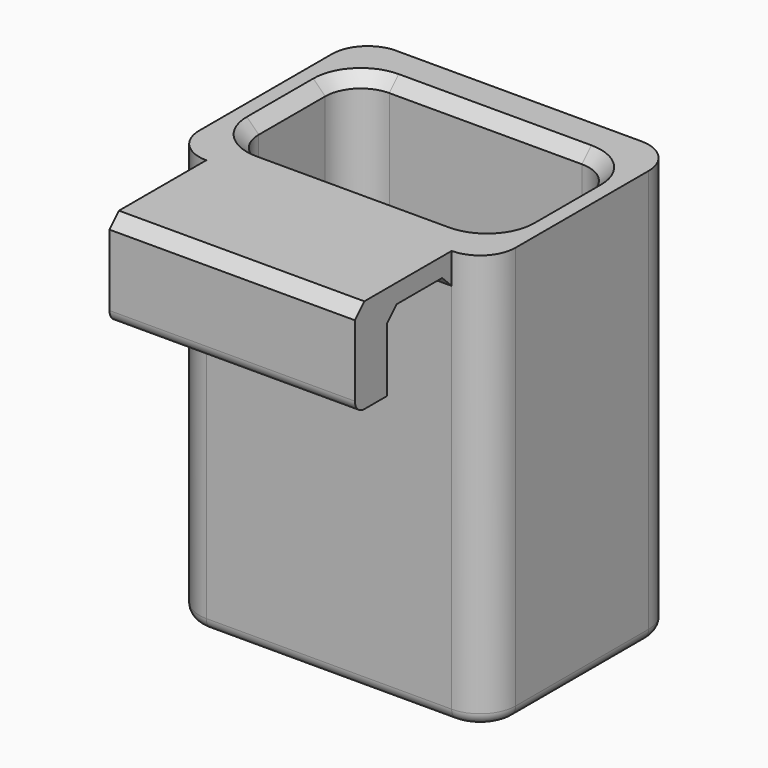
from build123d import *

# Parameters (mm, degrees)
F0_W          = 133.4117650986
F0_H          = 100
F0_W_2        = 111.1764758825
F0_H_2        = 65
F1_DEPTH      = 175
F2_DEPTH      = 2
F3_R          = 15
F4_W          = 103.4117650986
F4_H          = 34
F5_DEPTH      = 8
F4_H_2        = 17
F6_DEPTH      = 40
F7_SIZE       = 5
F8_SIZE       = 5
F9_R          = 5
F10_R         = 5
F12_DEPTH     = 25
F13_T1_DEPTH  = 103.4117650986
F13_T3_DEPTH  = 70
F13_T6_ANGLE  = 90
F13_T8_ANGLE  = 90
F13_T10_ANGLE = 90
F13_T12_ANGLE = 90


# Not quite as in the source:
# - a fillet or chamfer that OpenCascade refuses, or shapes differently, is made with other operations: its cross-section is extruded or revolved along the edge and cut away or added


with BuildPart() as f1:
    # F0 (on Top) → F1 (new body)
    with BuildSketch(Plane.XY):
        Rectangle(F0_W, F0_H)
        Rectangle(F0_W_2, F0_H_2, mode=Mode.SUBTRACT)
    extrude(amount=F1_DEPTH)

    # F0 (on Top) → F2 (join)
    with BuildSketch(Plane.XY):
        Rectangle(F0_W_2, F0_H_2)
    extrude(amount=F2_DEPTH)

    # F3
    f3_edges = [f1.edges().sort_by_distance(p)[0] for p in [
        (66.705883, -50, 87.5),
        (66.705883, 50, 87.5),
        (-66.705883, -50, 87.5),
        (-66.705883, 50, 87.5),
        (55.588238, -32.5, 88.5),
        (-55.588238, -32.5, 88.5),
        (-55.588238, 32.5, 88.5),
        (55.588238, 32.5, 88.5),
    ]]
    fillet(f3_edges, radius=F3_R)

    # F4 (on face) → F5 (join)
    with BuildSketch(Plane.XY.offset(175)):
        with Locations((0, -67)):
            Rectangle(F4_W, F4_H)
    extrude(amount=-F5_DEPTH)

    # F4 (on face) → F6 (join)
    with BuildSketch(Plane.XY.offset(175)):
        with Locations((0, -92.5)):
            Rectangle(F4_W, F4_H_2)
    extrude(amount=-F6_DEPTH)

    # F7
    f7_edges = [f1.edges().sort_by_distance(p)[0] for p in [
        (0, -101, 175),
        (0, -84, 167),
        (0, -50, 167),
    ]]
    chamfer(f7_edges, length=F7_SIZE)

    # F8
    f8_edges = [f1.edges().sort_by_distance(p)[0] for p in [
        (-51.19484, -28.106602, 175),
        (-55.588238, 0, 175),
        (-51.19484, 28.106602, 175),
        (0, 32.5, 175),
        (51.19484, 28.106602, 175),
        (55.588238, 0, 175),
        (51.19484, -28.106602, 175),
        (0, -32.5, 175),
    ]]
    chamfer(f8_edges, length=F8_SIZE)

    # F9
    f9_edges = [f1.edges().sort_by_distance(p)[0] for p in [
        (0, 32.5, 2),
        (51.19484, 28.106602, 2),
        (-51.19484, 28.106602, 2),
        (55.588238, 0, 2),
        (-55.588238, 0, 2),
        (51.19484, -28.106602, 2),
        (-51.19484, -28.106602, 2),
        (0, -32.5, 2),
    ]]
    fillet(f9_edges, radius=F9_R)

    # F10
    f10_edges = [f1.edges().sort_by_distance(p)[0] for p in [
        (0, -101, 135),
    ]]
    fillet(f10_edges, radius=F10_R)

    # F11 (on Top) → F12 (cut)
    with BuildSketch(Plane.XY):
        with BuildLine():
            Line((4.7656208593, -11.166036129), (18.7343597096, -11.166036129))
            ThreePointArc((18.7343597096, -11.166036129), (11.7499902844, -4.1816667038), (4.7656208593, -11.166036129))
        make_face()
        with BuildLine():
            ThreePointArc((4.7656208593, -11.166036129), (11.7499902844, -18.1504055542), (18.7343597096, -11.166036129))
            Line((18.7343597096, -11.166036129), (4.7656208593, -11.166036129))
        make_face()
        with BuildLine():
            ThreePointArc((14.9149444799, 13.5657899082), (9.0519720688, 19.4287623192), (3.1889996578, 13.5657899082))
            Line((3.1889996578, 13.5657899082), (14.9149444799, 13.5657899082))
        make_face()
        with BuildLine():
            Line((14.9149444799, 13.5657899082), (3.1889996578, 13.5657899082))
            ThreePointArc((3.1889996578, 13.5657899082), (9.0519720688, 7.7028174971), (14.9149444799, 13.5657899082))
        make_face()
        with BuildLine():
            ThreePointArc((42.3675444587, 13.5657899082), (36.0321477056, 19.9011866613), (29.6967509524, 13.5657899082))
            Line((29.6967509524, 13.5657899082), (42.3675444587, 13.5657899082))
        make_face()
        with BuildLine():
            Line((42.3675444587, 13.5657899082), (29.6967509524, 13.5657899082))
            ThreePointArc((29.6967509524, 13.5657899082), (36.0321477056, 7.230393155), (42.3675444587, 13.5657899082))
        make_face()
        with BuildLine():
            Line((29.4939792554, -11.166036129), (40.7716342409, -11.166036129))
            ThreePointArc((40.7716342409, -11.166036129), (35.1328067482, -5.5272086363), (29.4939792554, -11.166036129))
        make_face()
        with BuildLine():
            ThreePointArc((29.4939792554, -11.166036129), (35.1328067482, -16.8048636217), (40.7716342409, -11.166036129))
            Line((40.7716342409, -11.166036129), (29.4939792554, -11.166036129))
        make_face()
        with BuildLine():
            Line((-44.5507267353, -11.166036129), (-29.0779149297, -11.166036129))
            ThreePointArc((-29.0779149297, -11.166036129), (-36.8143208325, -3.4296302262), (-44.5507267353, -11.166036129))
        make_face()
        with BuildLine():
            ThreePointArc((-44.5507267353, -11.166036129), (-36.8143208325, -18.9024420318), (-29.0779149297, -11.166036129))
            Line((-29.0779149297, -11.166036129), (-44.5507267353, -11.166036129))
        make_face()
        with BuildLine():
            Line((-21.3590465179, -11.166036129), (-10.9000005135, -11.166036129))
            ThreePointArc((-10.9000005135, -11.166036129), (-16.1295235157, -5.9365131268), (-21.3590465179, -11.166036129))
        make_face()
        with BuildLine():
            ThreePointArc((-21.3590465179, -11.166036129), (-16.1295235157, -16.3955591312), (-10.9000005135, -11.166036129))
            Line((-10.9000005135, -11.166036129), (-21.3590465179, -11.166036129))
        make_face()
        with BuildLine():
            ThreePointArc((-12.6986786843, 13.5657899082), (-17.9282017052, 18.7953129291), (-23.1577247262, 13.5657899082))
            Line((-23.1577247262, 13.5657899082), (-12.6986786843, 13.5657899082))
        make_face()
        with BuildLine():
            Line((-12.6986786843, 13.5657899082), (-23.1577247262, 13.5657899082))
            ThreePointArc((-23.1577247262, 13.5657899082), (-17.9282017052, 8.3362668872), (-12.6986786843, 13.5657899082))
        make_face()
        with BuildLine():
            Line((-43.7775825475, 13.5657899082), (-36.1464346434, 13.5657899082))
            ThreePointArc((-36.1464346434, 13.5657899082), (-39.9620085955, 17.3813638602), (-43.7775825475, 13.5657899082))
        make_face()
        with BuildLine():
            ThreePointArc((-43.7775825475, 13.5657899082), (-39.9620085955, 9.7502159561), (-36.1464346434, 13.5657899082))
            Line((-36.1464346434, 13.5657899082), (-43.7775825475, 13.5657899082))
        make_face()
    extrude(amount=F12_DEPTH, mode=Mode.SUBTRACT)

    # F13: fillet of radius 5 on 16 edges, made by hand

    # F13_s2 → F13_t1 (cut)
    with BuildSketch(Plane.YZ.offset(-51.7058825493)):
        with BuildLine():
            ThreePointArc((45, 0), (48.5355339059, 1.4644660941), (50, 5))
            Line((50, 5), (50, 0))
            Line((50, 0), (45, 0))
        make_face()
        with BuildLine():
            ThreePointArc((-45, 0), (-48.5355339059, 1.4644660941), (-50, 5))
            Line((-50, 5), (-50, 0))
            Line((-50, 0), (-45, 0))
        make_face()
    extrude(amount=F13_T1_DEPTH, mode=Mode.SUBTRACT)

    # F13_s4 → F13_t3 (cut)
    with BuildSketch(Plane.XZ.offset(-35)):
        with BuildLine():
            ThreePointArc((61.7058825493, 0), (65.2414164552, 1.4644660941), (66.7058825493, 5))
            Line((66.7058825493, 5), (66.7058825493, 0))
            Line((66.7058825493, 0), (61.7058825493, 0))
        make_face()
        with BuildLine():
            ThreePointArc((-61.7058825493, 0), (-65.2414164552, 1.4644660941), (-66.7058825493, 5))
            Line((-66.7058825493, 5), (-66.7058825493, 0))
            Line((-66.7058825493, 0), (-61.7058825493, 0))
        make_face()
    extrude(amount=F13_T3_DEPTH, mode=Mode.SUBTRACT)

    # F13_s5 → F13_t6 (revolve, cut)
    with BuildSketch(Plane.YZ.offset(51.7058825493)):
        with BuildLine():
            ThreePointArc((45, 0), (48.5355339059, 1.4644660941), (50, 5))
            Line((50, 5), (50, 0))
            Line((50, 0), (45, 0))
        make_face()
    revolve(axis=Axis((51.7058825493, 35, 0), (0, 0, -1)), revolution_arc=F13_T6_ANGLE, mode=Mode.SUBTRACT)

    # F13_s7 → F13_t8 (revolve, cut)
    with BuildSketch(Plane.YZ.offset(-51.7058825493)):
        with BuildLine():
            ThreePointArc((45, 0), (48.5355339059, 1.4644660941), (50, 5))
            Line((50, 5), (50, 0))
            Line((50, 0), (45, 0))
        make_face()
    revolve(axis=Axis((-51.7058825493, 35, 0), (0, 0, 1)), revolution_arc=F13_T8_ANGLE, mode=Mode.SUBTRACT)

    # F13_s9 → F13_t10 (revolve, cut)
    with BuildSketch(Plane.XZ.offset(35)):
        with BuildLine():
            ThreePointArc((66.7058825493, 5), (65.2414164552, 1.4644660941), (61.7058825493, 0))
            Line((61.7058825493, 0), (66.7058825493, 0))
            Line((66.7058825493, 0), (66.7058825493, 5))
        make_face()
    revolve(axis=Axis((51.7058825493, -35, 0), (0, 0, -1)), revolution_arc=F13_T10_ANGLE, mode=Mode.SUBTRACT)

    # F13_s11 → F13_t12 (revolve, cut)
    with BuildSketch(Plane.XZ.offset(35)):
        with BuildLine():
            ThreePointArc((-61.7058825493, 0), (-65.2414164552, 1.4644660941), (-66.7058825493, 5))
            Line((-66.7058825493, 5), (-66.7058825493, 0))
            Line((-66.7058825493, 0), (-61.7058825493, 0))
        make_face()
    revolve(axis=Axis((-51.7058825493, -35, 0), (0, 0, 1)), revolution_arc=F13_T12_ANGLE, mode=Mode.SUBTRACT)

    # F13_s13 → F13_t14 (revolve, cut)
    with BuildSketch(Plane.XZ.offset(11.166036129)):
        with BuildLine():
            ThreePointArc((-48.5507267353, 0), (-46.3146587578, 0.527864045), (-44.5507267353, 2))
            Line((-44.5507267353, 2), (-44.5507267353, 0))
            Line((-44.5507267353, 0), (-48.5507267353, 0))
        make_face()
    revolve(axis=Axis((-36.8143208325, -11.166036129, 0), (0, 0, 1)), mode=Mode.SUBTRACT)

    # F13_s15 → F13_t16 (revolve, cut)
    with BuildSketch(Plane.XZ.offset(11.166036129)):
        with BuildLine():
            ThreePointArc((-25.3590465179, 0), (-23.1229785404, 0.527864045), (-21.3590465179, 2))
            Line((-21.3590465179, 2), (-21.3590465179, 0))
            Line((-21.3590465179, 0), (-25.3590465179, 0))
        make_face()
    revolve(axis=Axis((-16.1295235157, -11.166036129, 0), (0, 0, 1)), mode=Mode.SUBTRACT)

    # F13_s17 → F13_t18 (revolve, cut)
    with BuildSketch(Plane.XZ.offset(11.166036129)):
        with BuildLine():
            ThreePointArc((0.7656208593, 0), (3.0016888368, 0.527864045), (4.7656208593, 2))
            Line((4.7656208593, 2), (4.7656208593, 0))
            Line((4.7656208593, 0), (0.7656208593, 0))
        make_face()
    revolve(axis=Axis((11.7499902844, -11.166036129, 0), (0, 0, 1)), mode=Mode.SUBTRACT)

    # F13_s19 → F13_t20 (revolve, cut)
    with BuildSketch(Plane.XZ.offset(11.166036129)):
        with BuildLine():
            ThreePointArc((25.4939792554, 0), (27.7300472329, 0.527864045), (29.4939792554, 2))
            Line((29.4939792554, 2), (29.4939792554, 0))
            Line((29.4939792554, 0), (25.4939792554, 0))
        make_face()
    revolve(axis=Axis((35.1328067482, -11.166036129, 0), (0, 0, 1)), mode=Mode.SUBTRACT)

    # F13_s21 → F13_t22 (revolve, cut)
    with BuildSketch(Plane.XZ.offset(-13.5657899082)):
        with BuildLine():
            ThreePointArc((-47.7775825475, 0), (-45.54151457, 0.527864045), (-43.7775825475, 2))
            Line((-43.7775825475, 2), (-43.7775825475, 0))
            Line((-43.7775825475, 0), (-47.7775825475, 0))
        make_face()
    revolve(axis=Axis((-39.9620085955, 13.5657899082, 0), (0, 0, 1)), mode=Mode.SUBTRACT)

    # F13_s23 → F13_t24 (revolve, cut)
    with BuildSketch(Plane.XZ.offset(-13.5657899082)):
        with BuildLine():
            ThreePointArc((-27.1577247262, 0), (-24.9216567487, 0.527864045), (-23.1577247262, 2))
            Line((-23.1577247262, 2), (-23.1577247262, 0))
            Line((-23.1577247262, 0), (-27.1577247262, 0))
        make_face()
    revolve(axis=Axis((-17.9282017052, 13.5657899082, 0), (0, 0, 1)), mode=Mode.SUBTRACT)

    # F13_s25 → F13_t26 (revolve, cut)
    with BuildSketch(Plane.XZ.offset(-13.5657899082)):
        with BuildLine():
            ThreePointArc((-0.8110003422, 0), (1.4250676353, 0.527864045), (3.1889996578, 2))
            Line((3.1889996578, 2), (3.1889996578, 0))
            Line((3.1889996578, 0), (-0.8110003422, 0))
        make_face()
    revolve(axis=Axis((9.0519720688, 13.5657899082, 0), (0, 0, 1)), mode=Mode.SUBTRACT)

    # F13_s27 → F13_t28 (revolve, cut)
    with BuildSketch(Plane.XZ.offset(-13.5657899082)):
        with BuildLine():
            ThreePointArc((25.6967509524, 0), (27.9328189299, 0.527864045), (29.6967509524, 2))
            Line((29.6967509524, 2), (29.6967509524, 0))
            Line((29.6967509524, 0), (25.6967509524, 0))
        make_face()
    revolve(axis=Axis((36.0321477056, 13.5657899082, 0), (0, 0, 1)), mode=Mode.SUBTRACT)


solid = f1.part
